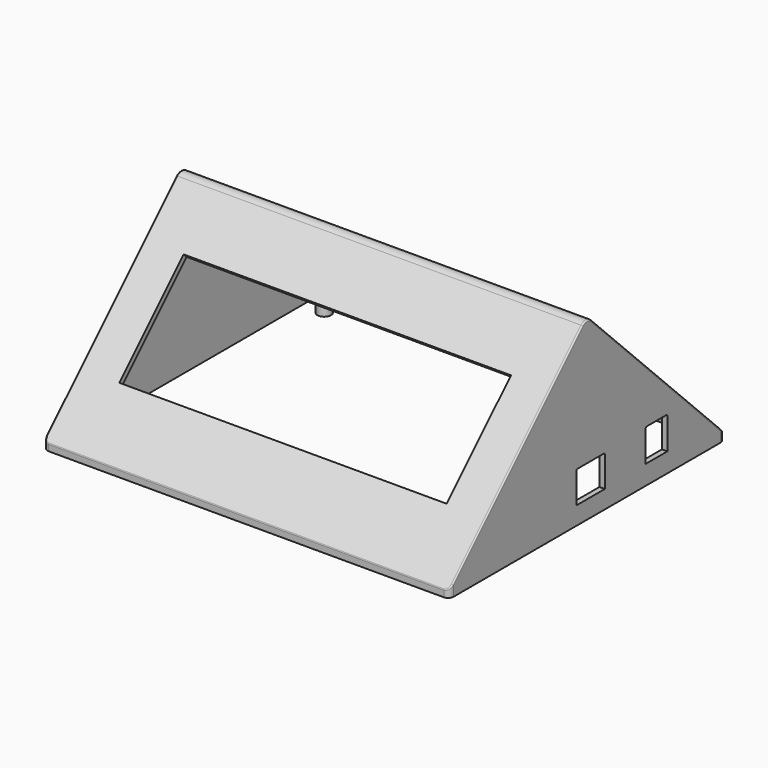
from build123d import *

# Parameters (mm, degrees)
F1_DEPTH  = 150
F2_T      = -2
F4_W      = 121
F4_H      = 42
F5_DEPTH  = 3
F6_R      = 3
F8_R      = 2.5
F8_R_2    = 1.5
F10_R     = 2.5
F10_R_2   = 1.25
F11_REACH = 69.4690374315
F12_W     = 150
F12_H     = 127.2792206136
F12_W_2   = 146
F12_H_2   = 121.6223663641
F13_DEPTH = 2.5
F14_R     = 2.5
F14_R_2   = 1.25
F16_R     = 2
F17_R     = 0.5
F7_W      = 10
F7_H      = 12
F7_W_2    = 13.1
F7_H_2    = 11.7
F18_DEPTH = 3
F19_R     = 0.5
F20_R     = 0.5
F21_R     = 6.5
F22_DEPTH = 2.5
F23_R     = 2.5
F23_R_2   = 1.25
F24_DEPTH = 2.5
F25_R     = 2.5
F26_DEPTH = 1.5
F27_R     = 3


with BuildPart() as f1:
    # F0 (on Right) → F1 (new body)
    with BuildSketch(Plane.YZ):
        Polygon((63.6396103068, 63.6396103068), (0, 0), (127.2792206136, 0), align=None)
    extrude(amount=F1_DEPTH)

    # F2
    f2_openings = [f1.faces().sort_by_distance(p)[0] for p in [
        (75, 63.63961, 0),
    ]]
    offset(amount=F2_T, openings=f2_openings)

    # F4 (on offset) → F5 (cut)
    with BuildSketch(Plane(origin=(0, 0, 0), x_dir=(1, 0, 0), z_dir=(0, -0.7071067812, 0.7071067812))):
        with Locations((75, 45)):
            Rectangle(F4_W, F4_H)
    extrude(amount=-F5_DEPTH, mode=Mode.SUBTRACT)

    # F6
    f6_edges = [f1.edges().sort_by_distance(p)[0] for p in [
        (75, 63.63961, 63.63961),
    ]]
    fillet(f6_edges, radius=F6_R)

    # F8 (on face) → F9 (join, up to the last surface of F1)
    with BuildSketch(Plane(origin=(0, 0, 0), x_dir=(1, 0, 0), z_dir=(0, 0, -1))):
        with Locations((10, -10)):
            Circle(F8_R)
        with Locations((10, -10)):
            Circle(F8_R_2, mode=Mode.SUBTRACT)
    extrude(until=Until.LAST, dir=(0, 0, 1))

    f11_end = Plane(origin=(75.2423938978, 33.320661552, 30.4922344273), x_dir=(0, 0.7071067812, 0.7071067812), z_dir=(0, 0.7071067812, -0.7071067812))
    # F10 (on face) → F11 (join, up to a plane its end follows)
    with BuildSketch(Plane(origin=(0, 0, 0), x_dir=(1, 0, 0), z_dir=(0, 0, -1))):
        with Locations((10, -10)):
            Circle(F10_R)
        with Locations((10, -10)):
            Circle(F10_R_2, mode=Mode.SUBTRACT)
        with Locations((140, -10)):
            Circle(F10_R)
        with Locations((140, -10)):
            Circle(F10_R_2, mode=Mode.SUBTRACT)
    f11_long = extrude(amount=-F11_REACH, mode=Mode.PRIVATE)
    add(split(f11_long, bisect_by=f11_end, keep=Keep.TOP, mode=Mode.PRIVATE))

    # F12 (on face) → F13 (join)
    with BuildSketch(Plane(origin=(0, 0, 0), x_dir=(1, 0, 0), z_dir=(0, 0, -1))):
        with Locations((75, -63.6396103068)):
            Rectangle(F12_W, F12_H)
        with Locations((75, -63.6396103068)):
            Rectangle(F12_W_2, F12_H_2, mode=Mode.SUBTRACT)
    extrude(amount=F13_DEPTH)

    # F14 (on Top) → F15 (join, up to the next surface of F1)
    with BuildSketch(Plane.XY):
        with Locations((140, 117.279)):
            Circle(F14_R)
        with Locations((140, 117.279)):
            Circle(F14_R_2, mode=Mode.SUBTRACT)
        with Locations((10, 117.279)):
            Circle(F14_R)
        with Locations((10, 117.279)):
            Circle(F14_R_2, mode=Mode.SUBTRACT)
    extrude(until=Until.NEXT)

    # F16
    f16_edges = [f1.edges().sort_by_distance(p)[0] for p in [
        (150, 127.279221, -1.25),
        (150, 0, -1.25),
        (0, 0, -1.25),
        (0, 127.279221, -1.25),
    ]]
    fillet(f16_edges, radius=F16_R)

    # F17
    f17_edges = [f1.edges().sort_by_distance(p)[0] for p in [
        (0, 31.759145, 31.759145),
    ]]
    fillet(f17_edges, radius=F17_R)

    # F7 (on face) → F18 (cut)
    with BuildSketch(Plane.YZ.offset(150)):
        with Locations((95.7792206136, 10.65)):
            Rectangle(F7_W, F7_H)
        with Locations((65.3223664939, 10.0139604606)):
            Rectangle(F7_W_2, F7_H_2)
    extrude(amount=-F18_DEPTH, mode=Mode.SUBTRACT)

    # F19
    f19_edges = [f1.edges().sort_by_distance(p)[0] for p in [
        (149, 90.779221, 16.65),
        (149, 100.779221, 16.65),
    ]]
    fillet(f19_edges, radius=F19_R)

    # F20
    f20_edges = [f1.edges().sort_by_distance(p)[0] for p in [
        (149, 71.872366, 15.86396),
        (149, 58.772366, 15.86396),
    ]]
    fillet(f20_edges, radius=F20_R)

    # F21 (on face) → F22 (cut)
    with BuildSketch(Plane(origin=(0, 0, 0), x_dir=(0, -1, 0), z_dir=(-1, 0, 0))):
        with Locations((-64, 47.5)):
            Circle(F21_R)
    extrude(amount=-F22_DEPTH, mode=Mode.SUBTRACT)

    # F23 (on face) → F24 (join)
    with BuildSketch(Plane(origin=(0, 0, 0), x_dir=(1, 0, 0), z_dir=(0, 0, -1))):
        with Locations((10, -10)):
            Circle(F23_R)
        with Locations((10, -10)):
            Circle(F23_R_2, mode=Mode.SUBTRACT)
        with Locations((140, -10)):
            Circle(F23_R)
        with Locations((140, -10)):
            Circle(F23_R_2, mode=Mode.SUBTRACT)
        with Locations((10, -117.279)):
            Circle(F23_R)
        with Locations((10, -117.279)):
            Circle(F23_R_2, mode=Mode.SUBTRACT)
        with Locations((140, -117.279)):
            Circle(F23_R)
        with Locations((140, -117.279)):
            Circle(F23_R_2, mode=Mode.SUBTRACT)
    extrude(amount=F24_DEPTH)

    # F25 (on face) → F26 (cut)
    with BuildSketch(Plane(origin=(0, 0, 0), x_dir=(0, -1, 0), z_dir=(-1, 0, 0))):
        with Locations((-64, 32.5)):
            Circle(F25_R)
    extrude(amount=-F26_DEPTH, mode=Mode.SUBTRACT)

    # F27
    f27_edges = [f1.edges().sort_by_distance(p)[0] for p in [
        (75, 63.63961, 60.811183),
    ]]
    fillet(f27_edges, radius=F27_R)


solid = f1.part
